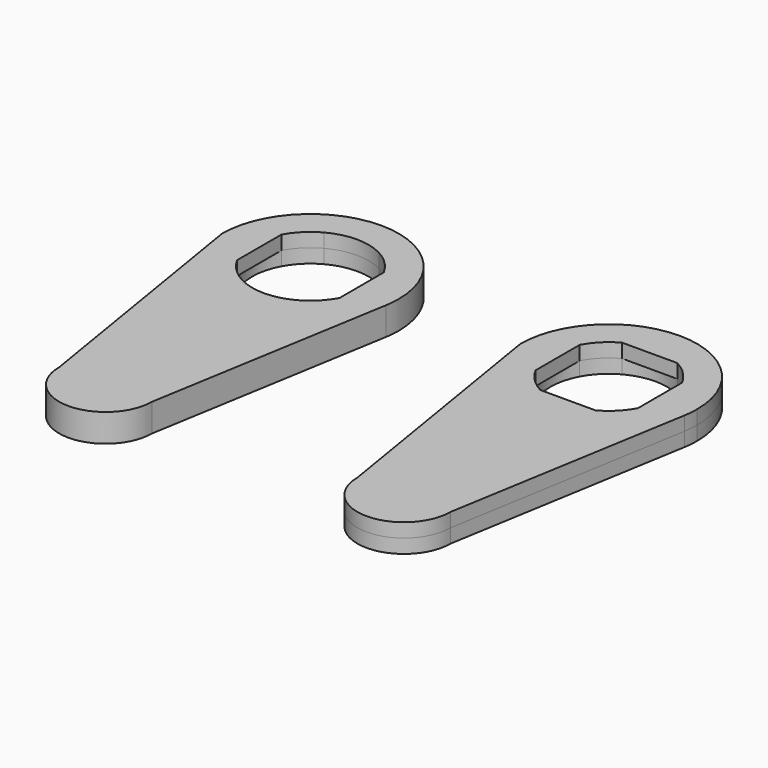
from build123d import *
from build123d import SkipClean  # not in build123d's __all__

# Parameters (mm, degrees)
F1_DEPTH = 3
F2_DEPTH = 3
F4_DEPTH = 25
F6_DEPTH = 25


with BuildPart() as f1:
    # F0 (on Top) → F1 (new body)
    with BuildSketch(Plane.XY):
        with BuildLine():
            ThreePointArc((18.7358645414, -3.1571157542), (18.9338509856, -1.5840728697), (19, 0))
            ThreePointArc((19, 0), (0, 19), (-19, 0))
            Line((-19, 0), (-18.00901481, -6.0560206053))
            ThreePointArc((-18.00901481, -6.0560206053), (1.4943192319, -18.9411459535), (18.7358645414, -3.1571157542))
        make_face()
        with BuildLine():
            Line((-11, 5.9371710435), (-11, 11))
            Line((-11, 11), (-5.9371710435, 11))
            ThreePointArc((-5.9371710435, 11), (0, 12.5), (5.9371710435, 11))
            Line((5.9371710435, 11), (11, 11))
            Line((11, 11), (11, 5.9371710435))
            ThreePointArc((11, 5.9371710435), (12.1191996435, 3.0618621785), (12.5, 0))
            ThreePointArc((12.5, 0), (12.1191996435, -3.0618621785), (11, -5.9371710435))
            Line((11, -5.9371710435), (11, -11))
            Line((11, -11), (5.9371710435, -11))
            ThreePointArc((5.9371710435, -11), (0, -12.5), (-5.9371710435, -11))
            Line((-5.9371710435, -11), (-11, -11))
            Line((-11, -11), (-11, -5.9371710435))
            ThreePointArc((-11, -5.9371710435), (-12.5, 0), (-11, 5.9371710435))
        make_face(mode=Mode.SUBTRACT)
        with BuildLine():
            Line((-18.00901481, -6.0560206053), (-19, 0))
            ThreePointArc((-19, 0), (-18.7506170751, -3.0682827941), (-18.00901481, -6.0560206053))
        make_face()
        with BuildLine():
            Line((10, -55), (18.7358645414, -3.1571157542))
            ThreePointArc((18.7358645414, -3.1571157542), (1.4943192319, -18.9411459535), (-18.00901481, -6.0560206053))
            Line((-18.00901481, -6.0560206053), (-10, -55))
            ThreePointArc((-10, -55), (0, -45), (10, -55))
        make_face()
        with BuildLine():
            ThreePointArc((-10, -55), (0, -65), (10, -55))
            ThreePointArc((10, -55), (0, -45), (-10, -55))
        make_face()
        with BuildLine():
            Line((-5.9371710435, 11), (-11, 11))
            Line((-11, 11), (-11, 5.9371710435))
            ThreePointArc((-11, 5.9371710435), (-8.8388347648, 8.8388347648), (-5.9371710435, 11))
        make_face()
        with BuildLine():
            ThreePointArc((5.9371710435, 11), (0, 12.5), (-5.9371710435, 11))
            Line((-5.9371710435, 11), (5.9371710435, 11))
        make_face()
        with BuildLine():
            Line((11, 11), (5.9371710435, 11))
            ThreePointArc((5.9371710435, 11), (8.8388347648, 8.8388347648), (11, 5.9371710435))
            Line((11, 5.9371710435), (11, 11))
        make_face()
        with BuildLine():
            Line((11, -11), (11, -5.9371710435))
            ThreePointArc((11, -5.9371710435), (8.8388347648, -8.8388347648), (5.9371710435, -11))
            Line((5.9371710435, -11), (11, -11))
        make_face()
        with BuildLine():
            ThreePointArc((12.5, 0), (12.1191996435, 3.0618621785), (11, 5.9371710435))
            Line((11, 5.9371710435), (11, -5.9371710435))
            ThreePointArc((11, -5.9371710435), (12.1191996435, -3.0618621785), (12.5, 0))
        make_face()
        with BuildLine():
            ThreePointArc((-5.9371710435, -11), (-8.8388347648, -8.8388347648), (-11, -5.9371710435))
            Line((-11, -5.9371710435), (-11, -11))
            Line((-11, -11), (-5.9371710435, -11))
        make_face()
        with BuildLine():
            Line((5.9371710435, -11), (-5.9371710435, -11))
            ThreePointArc((-5.9371710435, -11), (0, -12.5), (5.9371710435, -11))
        make_face()
        with BuildLine():
            Line((-11, -5.9371710435), (-11, 5.9371710435))
            ThreePointArc((-11, 5.9371710435), (-12.5, 0), (-11, -5.9371710435))
        make_face()
    extrude(amount=F1_DEPTH)

    # F0 (on Top) → F2 (join)
    with BuildSketch(Plane.XY):
        with BuildLine():
            ThreePointArc((18.7358645414, -3.1571157542), (18.9338509856, -1.5840728697), (19, 0))
            ThreePointArc((19, 0), (0, 19), (-19, 0))
            Line((-19, 0), (-18.00901481, -6.0560206053))
            ThreePointArc((-18.00901481, -6.0560206053), (1.4943192319, -18.9411459535), (18.7358645414, -3.1571157542))
        make_face()
        with BuildLine():
            Line((-11, 5.9371710435), (-11, 11))
            Line((-11, 11), (-5.9371710435, 11))
            ThreePointArc((-5.9371710435, 11), (0, 12.5), (5.9371710435, 11))
            Line((5.9371710435, 11), (11, 11))
            Line((11, 11), (11, 5.9371710435))
            ThreePointArc((11, 5.9371710435), (12.1191996435, 3.0618621785), (12.5, 0))
            ThreePointArc((12.5, 0), (12.1191996435, -3.0618621785), (11, -5.9371710435))
            Line((11, -5.9371710435), (11, -11))
            Line((11, -11), (5.9371710435, -11))
            ThreePointArc((5.9371710435, -11), (0, -12.5), (-5.9371710435, -11))
            Line((-5.9371710435, -11), (-11, -11))
            Line((-11, -11), (-11, -5.9371710435))
            ThreePointArc((-11, -5.9371710435), (-12.5, 0), (-11, 5.9371710435))
        make_face(mode=Mode.SUBTRACT)
        with BuildLine():
            Line((-5.9371710435, 11), (-11, 11))
            Line((-11, 11), (-11, 5.9371710435))
            ThreePointArc((-11, 5.9371710435), (-8.8388347648, 8.8388347648), (-5.9371710435, 11))
        make_face()
        with BuildLine():
            Line((11, 11), (5.9371710435, 11))
            ThreePointArc((5.9371710435, 11), (8.8388347648, 8.8388347648), (11, 5.9371710435))
            Line((11, 5.9371710435), (11, 11))
        make_face()
        with BuildLine():
            Line((11, -11), (11, -5.9371710435))
            ThreePointArc((11, -5.9371710435), (8.8388347648, -8.8388347648), (5.9371710435, -11))
            Line((5.9371710435, -11), (11, -11))
        make_face()
        with BuildLine():
            ThreePointArc((-5.9371710435, -11), (-8.8388347648, -8.8388347648), (-11, -5.9371710435))
            Line((-11, -5.9371710435), (-11, -11))
            Line((-11, -11), (-5.9371710435, -11))
        make_face()
        with BuildLine():
            Line((10, -55), (18.7358645414, -3.1571157542))
            ThreePointArc((18.7358645414, -3.1571157542), (1.4943192319, -18.9411459535), (-18.00901481, -6.0560206053))
            Line((-18.00901481, -6.0560206053), (-10, -55))
            ThreePointArc((-10, -55), (0, -45), (10, -55))
        make_face()
        with BuildLine():
            ThreePointArc((-10, -55), (0, -65), (10, -55))
            ThreePointArc((10, -55), (0, -45), (-10, -55))
        make_face()
    with SkipClean():  # cleaning this boolean's faces spoils the solid; the shape is the same uncleaned
        extrude(amount=-F2_DEPTH)

    # F3: union 

    # F4 (cut): a face of the model
    f4_faces = [f1.faces().sort_by_distance(p)[0] for p in [
        (-18.6030068603, -3.0441283953, 0),
    ]]
    with SkipClean():  # cleaning this boolean's faces spoils the solid; the shape is the same uncleaned
        extrude(f4_faces, amount=-F4_DEPTH, mode=Mode.SUBTRACT)


with BuildPart() as f5_1:
    # F5: copy of F1
    add(f1.part.moved(Location((-64.1, 0, 0))), clean=False)

    # F6 (cut): faces of the model
    f6_faces = [f5_1.faces().sort_by_distance(p)[0] for p in [
        (-64.1, 11.6031968432, 0),
        (-64.1, -11.6031968432, 0),
    ]]
    extrude(f6_faces, amount=-F6_DEPTH, mode=Mode.SUBTRACT)


solid = Compound([f1.part, f5_1.part])
